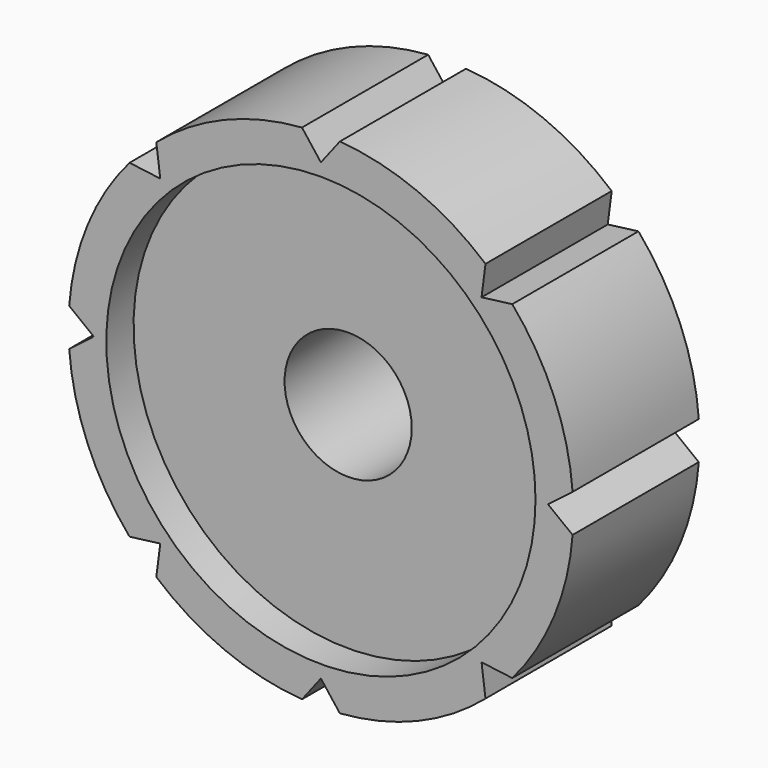
from build123d import *

# Parameters (mm, degrees)
F0_R            = 40
F1_DEPTH        = 25
F3_DEPTH        = 25
F3_COPIES_COUNT = 8
F4_R            = 10.0757297648
F5_DEPTH        = 25
F7_DEPTH        = 5.4


# Not quite as in the source:
# - a pattern or mirror of a feature is missing from the dataset's text; its kind, count and spacing are read off the source's solid


with BuildPart() as f1:
    # F0 (on Front) → F1 (new body)
    with BuildSketch(Plane.XZ):
        Circle(F0_R)
    extrude(amount=F1_DEPTH)

    # F2 (on face) → F3 (cut)
    with BuildSketch(Plane.XZ.offset(25)):
        with BuildLine():
            ThreePointArc((0, 40), (-1.5010572917, 39.971825415), (-3, 39.8873413504))
            Line((-3, 39.8873413504), (0, 36))
            Line((0, 36), (0, 40))
        make_face()
        with BuildLine():
            Line((0, 36), (3, 39.8873413504))
            ThreePointArc((3, 39.8873413504), (1.5010572917, 39.971825415), (0, 40))
            Line((0, 40), (0, 36))
        make_face()
    f3 = extrude(amount=-F3_DEPTH, mode=Mode.SUBTRACT)

    # F3_copies: F3 ×8 about axis
    f3_copies_axis = Axis((0, 0, 0), (0, 1, 0))
    for i in range(1, F3_COPIES_COUNT):
        add(f3.rotate(f3_copies_axis, i * 360 / F3_COPIES_COUNT), mode=Mode.SUBTRACT)

    # F4 (on face) → F5 (cut)
    with BuildSketch(Plane.XZ.offset(25)):
        Circle(F4_R)
    extrude(amount=-F5_DEPTH, mode=Mode.SUBTRACT)

    # F6 (on face) → F7 (cut)
    with BuildSketch(Plane.XZ.offset(25)):
        with BuildLine():
            ThreePointArc((0, 34.0096793756), (-24.0484749125, -24.0484749125), (34.0096793756, 0))
            ThreePointArc((34.0096793756, 0), (24.0484749125, 24.0484749125), (0, 34.0096793756))
        make_face()
    extrude(amount=-F7_DEPTH, mode=Mode.SUBTRACT)


solid = f1.part
